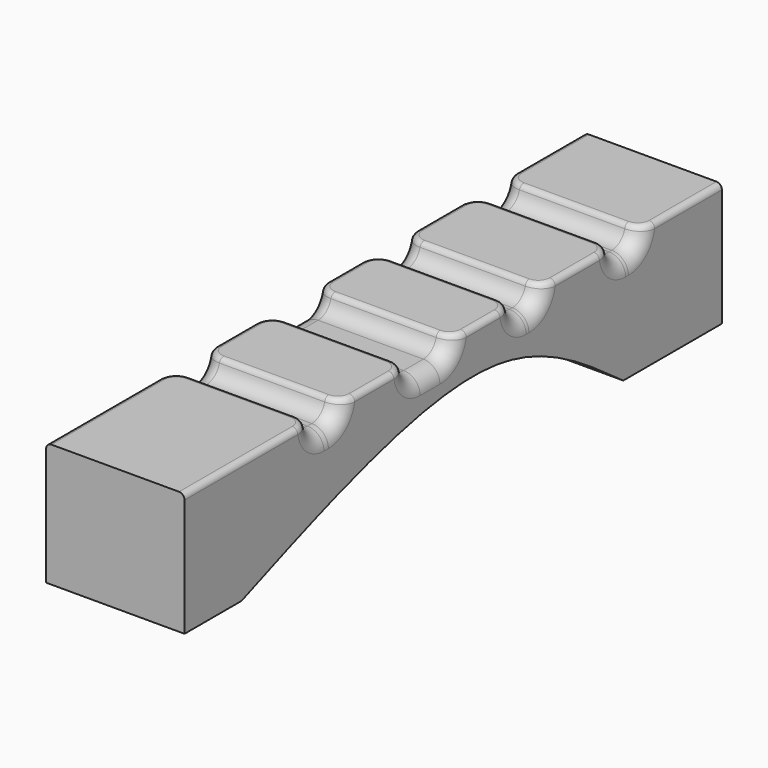
from build123d import *

# Parameters (mm, degrees)
F1_DEPTH = 25
F2_W     = 25
F2_H     = 6.9918222725
F2_H_2   = 10.4526877403
F2_H_3   = 6.6238343716
F2_H_4   = 6.623826921
F3_DEPTH = 3
F4_F1_R  = 2.9999
F4_F2_R  = 3
F5_R     = 1


# Not quite as in the source:
# - a fillet or chamfer is up to 0.001 mm smaller than in the source, because OpenCascade refuses the exact size


with BuildPart() as f1:
    # F0 (on Right) → F1 (new body)
    with BuildSketch(Plane.YZ):
        with BuildLine():
            Line((0, 22.2572330385), (0, 0))
            Line((0, 0), (12.8407105803, 0))
            add(Edge.make_bspline(
                [(99.0161448717, 0), (90.0391263574, 6.5433116329), (69.1199405475, 21.7912195704), (33.2931848707, 7.9191623318), (12.8407105803, 0)],
                knots=[0, 0, 0, 0, 0.429128485, 1, 1, 1, 1], degree=3))
            Line((99.0161448717, 0), (121.2733760476, 0))
            Line((121.2733760476, 0), (121.2733760476, 22.2572330385))
            Line((121.2733760476, 22.2572330385), (0, 22.2572330385))
        make_face()
    extrude(amount=-F1_DEPTH)

    # F2 (on face) → F3 (cut)
    with BuildSketch(Plane.XY.offset(22.2572330385)):
        with Locations((-12.5, 31.9684613496)):
            Rectangle(F2_W, F2_H)
        with Locations((-12.5, 55.4103441536)):
            Rectangle(F2_W, F2_H_2)
        with Locations((-12.5, 77.4153098464)):
            Rectangle(F2_W, F2_H_3)
        with Locations((-12.5, 99.8627357185)):
            Rectangle(F2_W, F2_H_4)
    extrude(amount=-F3_DEPTH, mode=Mode.SUBTRACT)

    # F4: fillet of radius 3 on 16 edges, made by hand

    # F4_f1 (radius 3 in the source; OpenCascade refuses exactly that, so slightly less here)
    f4_f1_edges = [f1.edges().sort_by_distance(p)[0] for p in [
        (-12.5, 28.4725502133, 19.2572330385),
        (-12.5, 35.4643724859, 19.2572330385),
        (-12.5, 50.1840002835, 19.2572330385),
        (-12.5, 60.6366880238, 19.2572330385),
        (-12.5, 74.1033926606, 19.2572330385),
        (-12.5, 80.7272270322, 19.2572330385),
        (-12.5, 96.550822258, 19.2572330385),
        (-12.5, 103.174649179, 19.2572330385),
    ]]
    fillet(f4_f1_edges, radius=F4_F1_R)

    # F4_f2
    f4_f2_edges = [f1.edges().sort_by_distance(p)[0] for p in [
        (-25, 31.9684613496, 19.2572330385),
        (0, 31.9684613496, 19.2572330385),
        (-25, 55.4103441536, 19.2572330385),
        (0, 55.4103441536, 19.2572330385),
        (-25, 77.4153098464, 19.2572330385),
        (0, 77.4153098464, 19.2572330385),
        (-25, 99.8627357185, 19.2572330385),
        (0, 99.8627357185, 19.2572330385),
        (0, 97.4294726251, 20.1358834057),
        (0, 102.2959988119, 20.1358834057),
        (-25, 102.2959988119, 20.1358834057),
        (-25, 97.4294726251, 20.1358834057),
        (0, 74.9820430277, 20.1358834057),
        (0, 79.8485766651, 20.1358834057),
        (-25, 79.8485766651, 20.1358834057),
        (-25, 74.9820430277, 20.1358834057),
        (0, 51.0626506506, 20.1358834057),
        (0, 59.7580376567, 20.1358834057),
        (-25, 59.7580376567, 20.1358834057),
        (-25, 51.0626506506, 20.1358834057),
        (0, 29.3512005805, 20.1358834057),
        (0, 34.5857221188, 20.1358834057),
        (-25, 34.5857221188, 20.1358834057),
        (-25, 29.3512005805, 20.1358834057),
    ]]
    fillet(f4_f2_edges, radius=F4_F2_R)

    # F5
    f5_edges = [f1.edges().sort_by_distance(p)[0] for p in [
        (0, 12.736275, 22.257233),
        (0, 42.824186, 22.257233),
        (0, 113.724013, 22.257233),
        (0, 67.37004, 22.257233),
        (0, 88.639025, 22.257233),
        (-25, 12.736275, 22.257233),
        (-25, 42.824186, 22.257233),
        (-25, 113.724013, 22.257233),
        (-25, 67.37004, 22.257233),
        (-25, 88.639025, 22.257233),
    ]]
    fillet(f5_edges, radius=F5_R)


solid = f1.part
